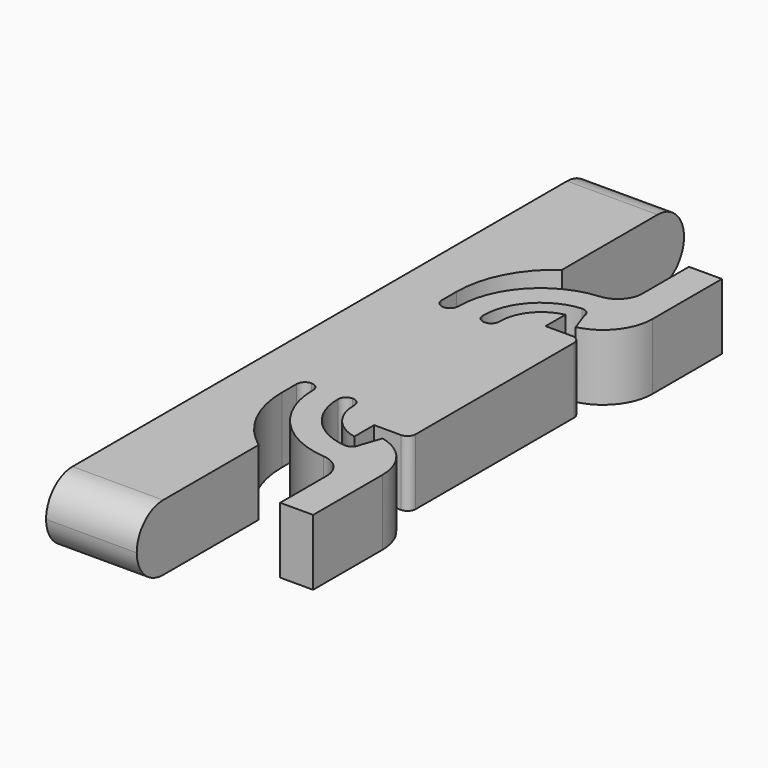
from build123d import *

# Parameters (mm, degrees)
F0_W          = 4
F0_H          = 8
F0_H_2        = 2
F0_W_2        = 5.5
F0_H_3        = 3.5
F0_W_3        = 4.25
F0_H_4        = 26
F1_DEPTH      = 8
F2_R          = 3.99999
F3_T1_DEPTH   = 37.8956518578
F4_T1_DEPTH   = 21.1532650868
F5_T1_DEPTH   = 21.1532650868
F6_R          = 1.75
F7_DEPTH      = 10
F8_T1_DEPTH   = 32.4948974279
F9_R          = 7
F10_R         = 10
F11_T1_DEPTH  = 8
F12_R         = 3
F13_T1_DEPTH  = 8
F13_T3_DEPTH  = 8
F13_T5_DEPTH  = 8
F13_T7_DEPTH  = 8
F13_T9_DEPTH  = 8
F13_T11_DEPTH = 8
F13_T13_DEPTH = 8
F13_T15_DEPTH = 8
F13_T17_DEPTH = 8
F13_T19_DEPTH = 8
F13_T21_DEPTH = 13
F13_T23_DEPTH = 13


# Not quite as in the source:
# - a fillet or chamfer that OpenCascade refuses, or shapes differently, is made with other operations: its cross-section is extruded or revolved along the edge and cut away or added
# - two fillets or chamfers of one size are made in one step
# - a fillet or chamfer is up to 0.001 mm smaller than in the source, because OpenCascade refuses the exact size


with BuildPart() as f1:
    # F0 (on Top) → F1 (new body)
    with BuildSketch(Plane.XY):
        Polygon((0, 83), (0, 0), (11, 0), (11, 10), (11, 18.5), (6, 18.5), (6, 31.5), (8, 31.5), (11, 31.5), (13, 31.5), (13, 25.5), (17, 25.5), (17, 28.5), (17, 54.5), (17, 57.5), (13, 57.5), (13, 51.5), (11, 51.5), (8, 51.5), (6, 51.5), (6, 64.5), (11, 64.5), (11, 73), (11, 83), align=None)
        with Locations((22, 68.5)):
            Rectangle(F0_W, F0_H)
        with Locations((22, 63.5)):
            Rectangle(F0_W, F0_H_2)
        with Locations((21.25, 57.75)):
            Rectangle(F0_W_2, F0_H_3)
        with Locations((21.25, 25.25)):
            Rectangle(F0_W_2, F0_H_3)
        with Locations((22, 19.5)):
            Rectangle(F0_W, F0_H_2)
        with Locations((22, 14.5)):
            Rectangle(F0_W, F0_H)
        Polygon((11, 23.5), (11, 20.5), (20, 20.5), (24, 20.5), (24, 23.5), (18.5, 23.5), (17, 23.5), align=None)
        Polygon((8, 20.5), (11, 20.5), (11, 23.5), (11, 25.5), (11, 31.5), (8, 31.5), align=None)
        Polygon((11, 59.5), (11, 62.5), (8, 62.5), (8, 51.5), (11, 51.5), (11, 57.5), align=None)
        Polygon((20, 62.5), (11, 62.5), (11, 59.5), (17, 59.5), (18.5, 59.5), (24, 59.5), (24, 62.5), align=None)
        with Locations((19.125, 41.5)):
            Rectangle(F0_W_3, F0_H_4)
    extrude(amount=F1_DEPTH)

    # F2 (radius 4 in the source; OpenCascade refuses exactly that, so slightly less here)
    f2_edges = [f1.edges().sort_by_distance(p)[0] for p in [
        (5.5, 83, 8),
        (5.5, 0, 8),
        (5.5, 0, 0),
        (5.5, 83, 0),
    ]]
    fillet(f2_edges, radius=F2_R)

    # F3: fillet of radius 6 on 2 edges, made by hand

    # F3_s2 → F3_t1 (cut)
    with BuildSketch(Plane.XY.offset(-14.9478259289)):
        with BuildLine():
            ThreePointArc((24, 61.9791303716), (22.4158804332, 57.9171111692), (18.5, 56))
            Line((18.5, 56), (24, 56))
            Line((24, 56), (24, 61.9791303716))
        make_face()
        with BuildLine():
            ThreePointArc((24, 21.0208696284), (22.4158804332, 25.0828888308), (18.5, 27))
            Line((18.5, 27), (24, 27))
            Line((24, 27), (24, 21.0208696284))
        make_face()
    extrude(amount=F3_T1_DEPTH, mode=Mode.SUBTRACT)

    # F4: chamfer of 0.5 x 2.5 on 1 edges, made by hand

    # F4_s2 → F4_t1 (cut)
    with BuildSketch(Plane.XY.offset(-6.5766325434)):
        with BuildLine():
            Line((19.379363756, 56.0377654524), (18.466798813, 58.6304434947))
            Line((18.466798813, 58.6304434947), (18.416798813, 58.6304434947))
            ThreePointArc((18.416798813, 58.6304434947), (18.45, 57.3152217474), (18.45, 56))
            Line((18.45, 56), (18.5041666667, 55.9501739136))
            ThreePointArc((18.5041666667, 55.9501739136), (18.9421943049, 56.0029468158), (19.3905817774, 55.9890401407))
            Line((19.3905817774, 55.9890401407), (19.379363756, 56.0377654524))
        make_face()
    extrude(amount=F4_T1_DEPTH, mode=Mode.SUBTRACT)

    # F5: chamfer of 0.5 x 2.5 on 1 edges, made by hand

    # F5_s2 → F5_t1 (cut)
    with BuildSketch(Plane.XY.offset(-6.5766325434)):
        with BuildLine():
            Line((18.466798813, 24.3695565053), (19.379363756, 26.9622345476))
            Line((19.379363756, 26.9622345476), (19.3905817774, 27.0109598593))
            ThreePointArc((19.3905817774, 27.0109598593), (18.9421943049, 26.9970531842), (18.5041666667, 27.0498260864))
            Line((18.5041666667, 27.0498260864), (18.45, 27))
            ThreePointArc((18.45, 27), (18.45, 25.6847782526), (18.416798813, 24.3695565053))
            Line((18.416798813, 24.3695565053), (18.466798813, 24.3695565053))
        make_face()
    extrude(amount=F5_T1_DEPTH, mode=Mode.SUBTRACT)

    # F6 (on face) → F7 (cut)
    with BuildSketch(Plane(origin=(0, 0, 0), x_dir=(0, -1, 0), z_dir=(-1, 0, 0))):
        with Locations((-79, 4)):
            Circle(F6_R)
        with Locations((-4, 4)):
            Circle(F6_R)
    extrude(amount=-F7_DEPTH, mode=Mode.SUBTRACT)

    # F8: fillet of radius 5 on 2 edges, made by hand

    # F8_s2 → F8_t1 (cut)
    with BuildSketch(Plane.XY.offset(-12.2474487139)):
        with BuildLine():
            ThreePointArc((13, 52.6010205144), (14.1270166538, 55.7632981746), (17, 57.5))
            Line((17, 57.5), (13, 57.5))
            Line((13, 57.5), (13, 52.6010205144))
        make_face()
        with BuildLine():
            ThreePointArc((17, 25.5), (14.1270166538, 27.2367018254), (13, 30.3989794856))
            Line((13, 30.3989794856), (13, 25.5))
            Line((13, 25.5), (17, 25.5))
        make_face()
    extrude(amount=F8_T1_DEPTH, mode=Mode.SUBTRACT)

    # F9
    f9_edges = [f1.edges().sort_by_distance(p)[0] for p in [
        (11, 59.5, 4),
        (11, 23.5, 4),
    ]]
    fillet(f9_edges, radius=F9_R)

    # F10
    f10_edges = [f1.edges().sort_by_distance(p)[0] for p in [
        (8, 62.5, 4),
        (8, 20.5, 4),
    ]]
    fillet(f10_edges, radius=F10_R)

    # F11: fillet of radius 12 on 2 edges, made by hand

    # F11_s2 → F11_t1 (join)
    with BuildSketch(Plane.XY):
        with BuildLine():
            ThreePointArc((6, 54.7532056552), (7.322921748, 60.2304312302), (11, 64.5))
            Line((11, 64.5), (6, 64.5))
            Line((6, 64.5), (6, 54.7532056552))
        make_face()
        with BuildLine():
            ThreePointArc((11, 18.5), (7.322921748, 22.7695687698), (6, 28.2467943448))
            Line((6, 28.2467943448), (6, 18.5))
            Line((6, 18.5), (11, 18.5))
        make_face()
    extrude(amount=F11_T1_DEPTH)

    # F12
    f12_edges = [f1.edges().sort_by_distance(p)[0] for p in [
        (20, 62.5, 4),
        (20, 20.5, 4),
    ]]
    fillet(f12_edges, radius=F12_R)

    # F13: fillet of radius 1 on 12 edges, made by hand

    # F13_s2 → F13_t1 (join)
    with BuildSketch(Plane.XY):
        with BuildLine():
            ThreePointArc((8, 52.5), (7.7071067812, 51.7928932188), (7, 51.5))
            Line((7, 51.5), (8, 51.5))
            Line((8, 51.5), (8, 52.5))
        make_face()
    extrude(amount=F13_T1_DEPTH)

    # F13_s4 → F13_t3 (join)
    with BuildSketch(Plane.XY):
        with BuildLine():
            ThreePointArc((7, 51.5), (6.2928932188, 51.7928932188), (6, 52.5))
            Line((6, 52.5), (6, 51.5))
            Line((6, 51.5), (7, 51.5))
        make_face()
    extrude(amount=F13_T3_DEPTH)

    # F13_s6 → F13_t5 (join)
    with BuildSketch(Plane.XY):
        with BuildLine():
            ThreePointArc((18.5, 58.536115974), (18.1575199019, 59.2341109303), (17.4185535189, 59.4758096297))
            Line((17.4185535189, 59.4758096297), (17.4102471406, 59.575464053))
            ThreePointArc((17.4102471406, 59.575464053), (18, 59.6), (18.5, 59.6))
            Line((18.5, 59.6), (18.6, 59.5))
            ThreePointArc((18.6, 59.5), (18.6, 59.018057987), (18.5998382698, 58.5418010318))
            Line((18.5998382698, 58.5418010318), (18.5, 58.536115974))
        make_face()
    extrude(amount=F13_T5_DEPTH)

    # F13_s8 → F13_t7 (join)
    with BuildSketch(Plane.XY):
        with BuildLine():
            ThreePointArc((11, 52.5), (11.2928932188, 51.7928932188), (12, 51.5))
            Line((12, 51.5), (11, 51.5))
            Line((11, 51.5), (11, 52.5))
        make_face()
    extrude(amount=F13_T7_DEPTH)

    # F13_s10 → F13_t9 (join)
    with BuildSketch(Plane.XY):
        with BuildLine():
            ThreePointArc((13, 52.5), (12.7071067812, 51.7928932188), (12, 51.5))
            Line((12, 51.5), (13, 51.5))
            Line((13, 51.5), (13, 52.5))
        make_face()
    extrude(amount=F13_T9_DEPTH)

    # F13_s12 → F13_t11 (join)
    with BuildSketch(Plane.XY):
        with BuildLine():
            ThreePointArc((7, 31.5), (6.2928932188, 31.2071067812), (6, 30.5))
            Line((6, 30.5), (6, 31.5))
            Line((6, 31.5), (7, 31.5))
        make_face()
    extrude(amount=F13_T11_DEPTH)

    # F13_s14 → F13_t13 (join)
    with BuildSketch(Plane.XY):
        with BuildLine():
            ThreePointArc((7, 31.5), (7.7071067812, 31.2071067812), (8, 30.5))
            Line((8, 30.5), (8, 31.5))
            Line((8, 31.5), (7, 31.5))
        make_face()
    extrude(amount=F13_T13_DEPTH)

    # F13_s16 → F13_t15 (join)
    with BuildSketch(Plane.XY):
        with BuildLine():
            ThreePointArc((13, 30.5), (12.7071067812, 31.2071067812), (12, 31.5))
            Line((12, 31.5), (13, 31.5))
            Line((13, 31.5), (13, 30.5))
        make_face()
    extrude(amount=F13_T15_DEPTH)

    # F13_s18 → F13_t17 (join)
    with BuildSketch(Plane.XY):
        with BuildLine():
            ThreePointArc((11, 30.5), (11.2928932188, 31.2071067812), (12, 31.5))
            Line((12, 31.5), (11, 31.5))
            Line((11, 31.5), (11, 30.5))
        make_face()
    extrude(amount=F13_T17_DEPTH)

    # F13_s20 → F13_t19 (join)
    with BuildSketch(Plane.XY):
        with BuildLine():
            ThreePointArc((17.4185535189, 23.5241903703), (18.1575199019, 23.7658890697), (18.5, 24.463884026))
            Line((18.5, 24.463884026), (18.5998382698, 24.4581989682))
            ThreePointArc((18.5998382698, 24.4581989682), (18.6, 23.981942013), (18.6, 23.5))
            Line((18.6, 23.5), (18.5, 23.4))
            ThreePointArc((18.5, 23.4), (18, 23.4), (17.4102471406, 23.424535947))
            Line((17.4102471406, 23.424535947), (17.4185535189, 23.5241903703))
        make_face()
    extrude(amount=F13_T19_DEPTH)

    # F13_s22 → F13_t21 (cut)
    with BuildSketch(Plane.XY.offset(-2.5)):
        with BuildLine():
            ThreePointArc((20.25, 54.5), (20.9571067812, 54.2071067812), (21.25, 53.5))
            Line((21.25, 53.5), (21.25, 54.5))
            Line((21.25, 54.5), (20.25, 54.5))
        make_face()
    extrude(amount=F13_T21_DEPTH, mode=Mode.SUBTRACT)

    # F13_s24 → F13_t23 (cut)
    with BuildSketch(Plane.XY.offset(-2.5)):
        with BuildLine():
            ThreePointArc((21.25, 29.5), (20.9571067812, 28.7928932188), (20.25, 28.5))
            Line((20.25, 28.5), (21.25, 28.5))
            Line((21.25, 28.5), (21.25, 29.5))
        make_face()
    extrude(amount=F13_T23_DEPTH, mode=Mode.SUBTRACT)


solid = f1.part
